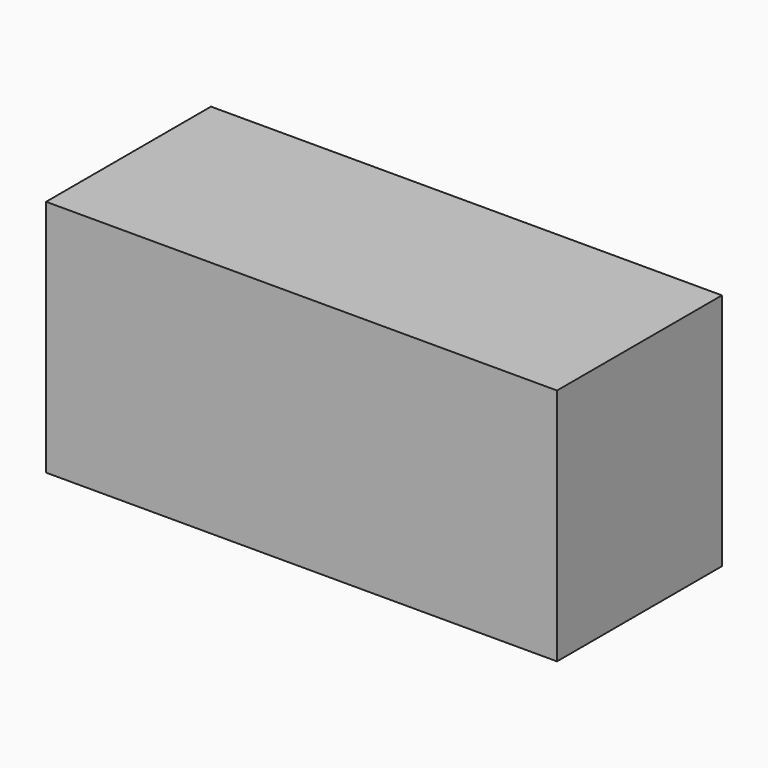
from build123d import *

# Parameters (mm, degrees)
F0_W       = 96.4113287628
F0_H       = 38.8907492161
F1_DEPTH   = 20
F2_R       = 6.9057023469
F1_FACE1_W = 96.4113287628
F1_FACE1_H = 38.8907492161
F3_DEPTH   = 25


with BuildPart() as f1:
    # F0 (on Top) → F1 (new body)
    with BuildSketch(Plane.XY):
        with Locations((-60.1103845984, 2.121495083)):
            Rectangle(F0_W, F0_H)
    extrude(amount=F1_DEPTH)

    # F2 (on face) + F1_face1 (on face) → F3 (join)
    with BuildSketch(Plane.XY.offset(20)):
        with Locations((-92.1053960919, 0)):
            Circle(F2_R)
    with BuildSketch(Plane(origin=(-60.1103845984, 2.121495083, 0), x_dir=(1, 0, 0), z_dir=(0, 0, -1))):
        Rectangle(F1_FACE1_W, F1_FACE1_H)
    extrude(amount=-F3_DEPTH, dir=(0, 0, 1))


solid = f1.part
